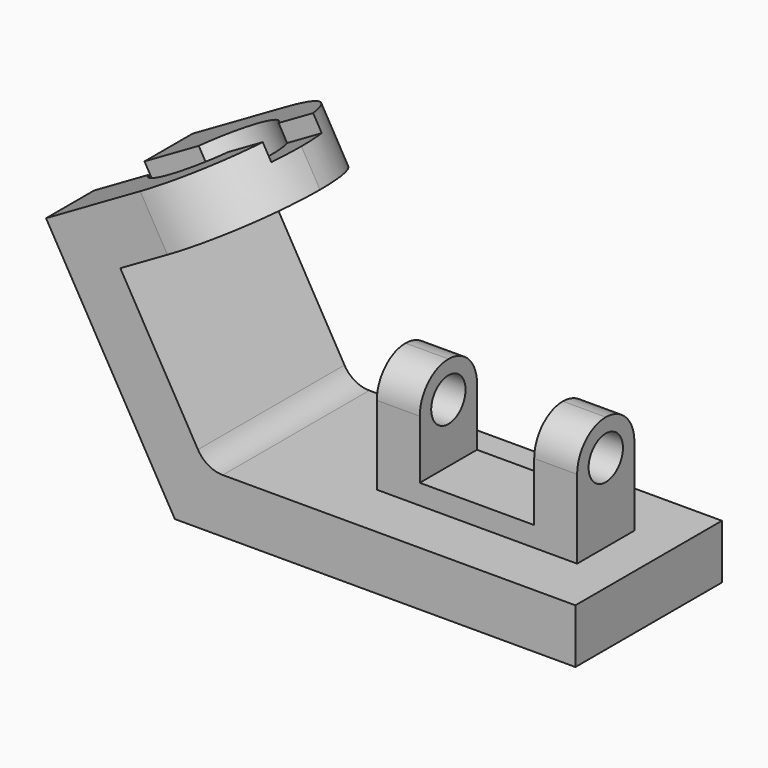
from build123d import *

# Parameters (mm, degrees)
F1_DEPTH  = 32
F2_DEPTH  = 12.5
F4_DEPTH  = 19
F5_R      = 10
F6_R      = 5
F7_DEPTH  = 19
F6_R_2    = 19.5
F8_DEPTH  = 12
F10_DEPTH = 6
F11_W     = 22
F11_H     = 56
F12_DEPTH = 6
F14_DEPTH = 70
F15_R     = 7.5
F16_DEPTH = 70


with BuildPart() as f1:
    # F0 (on Front) → F1 (new body, symmetric)
    with BuildSketch(Plane.XZ):
        Polygon((-45, 77.9422863406), (0, 0), (140, 0), (140, 19), (125, 19), (55, 19), (10.9696551146, 19), (-19.0455173281, 70.9878036687), (25.1217782649, 96.4878036687), (15.6217782649, 112.9422863406), align=None)
    extrude(amount=F1_DEPTH, both=True)

    # F0 (on Front) → F2 (join, symmetric)
    with BuildSketch(Plane.XZ):
        Polygon((55, 19), (125, 19), (125, 59), (110, 59), (110, 26), (70, 26), (70, 59), (55, 59), align=None)
    extrude(amount=F2_DEPTH, both=True)

    # F3 (on face) → F4 (cut, through all)
    with BuildSketch(Plane(origin=(-45, 0, 77.9422863406), x_dir=(0.8660254038, 0, 0.5), z_dir=(-0.5, 0, 0.8660254038))):
        with BuildLine():
            ThreePointArc((38, 32), (60.627416998, 22.627416998), (70, 0))
            Line((70, 0), (70, 32))
            Line((70, 32), (38, 32))
        make_face()
        with BuildLine():
            Line((70, -32), (70, 0))
            ThreePointArc((70, 0), (60.627416998, -22.627416998), (38, -32))
            Line((38, -32), (70, -32))
        make_face()
    extrude(amount=-F4_DEPTH, mode=Mode.SUBTRACT)

    # F5
    f5_edges = [f1.edges().sort_by_distance(p)[0] for p in [
        (10.969655, 0, 19),
    ]]
    fillet(f5_edges, radius=F5_R)

    # F6 (on face) → F7 (cut, through all)
    with BuildSketch(Plane(origin=(-45, 0, 77.9422863406), x_dir=(0.8660254038, 0, 0.5), z_dir=(-0.5, 0, 0.8660254038))):
        with Locations((38, 0)):
            Circle(F6_R)
    extrude(amount=-F7_DEPTH, mode=Mode.SUBTRACT)

    # F6 (on face) → F8 (cut)
    with BuildSketch(Plane(origin=(-45, 0, 77.9422863406), x_dir=(0.8660254038, 0, 0.5), z_dir=(-0.5, 0, 0.8660254038))):
        with Locations((38, 0)):
            Circle(F6_R_2)
        with Locations((38, 0)):
            Circle(F6_R, mode=Mode.SUBTRACT)
    extrude(amount=-F8_DEPTH, mode=Mode.SUBTRACT)

    # F9 (on face) → F10 (cut)
    with BuildSketch(Plane(origin=(-45, 0, 77.9422863406), x_dir=(0.8660254038, 0, 0.5), z_dir=(-0.5, 0, 0.8660254038))):
        with BuildLine():
            Line((21.8987578119, 11), (0, 11))
            Line((0, 11), (0, -11))
            Line((0, -11), (21.8987578119, -11))
            ThreePointArc((21.8987578119, -11), (18.5, 0), (21.8987578119, 11))
        make_face()
        with BuildLine():
            Line((68.0499584026, 11), (54.1012421881, 11))
            ThreePointArc((54.1012421881, 11), (56.630944993, 5.7565518035), (57.5, 0))
            ThreePointArc((57.5, 0), (56.630944993, -5.7565518035), (54.1012421881, -11))
            Line((54.1012421881, -11), (68.0499584026, -11))
            ThreePointArc((68.0499584026, -11), (70, 0), (68.0499584026, 11))
        make_face()
    extrude(amount=-F10_DEPTH, mode=Mode.SUBTRACT)

    # F11 (on face) → F12 (cut)
    with BuildSketch(Plane(origin=(0, 0, 0), x_dir=(0, -1, 0), z_dir=(-0.8660254038, 0, -0.5))):
        with Locations((0, 56)):
            Rectangle(F11_W, F11_H)
    extrude(amount=-F12_DEPTH, mode=Mode.SUBTRACT)

    # F13 (on face) → F14 (cut, through all)
    with BuildSketch(Plane.YZ.offset(125)):
        with BuildLine():
            ThreePointArc((-12.5, 46.5), (-8.8388347372, 55.3388347924), (7.81e-08, 59))
            Line((7.81e-08, 59), (-12.5, 59))
            Line((-12.5, 59), (-12.5, 46.5))
        make_face()
        with BuildLine():
            ThreePointArc((7.81e-08, 59), (8.8388347924, 55.3388347372), (12.5, 46.5))
            Line((12.5, 46.5), (12.5, 59))
            Line((12.5, 59), (7.81e-08, 59))
        make_face()
    extrude(amount=-F14_DEPTH, mode=Mode.SUBTRACT)

    # F15 (on face) → F16 (cut, through all)
    with BuildSketch(Plane.YZ.offset(125)):
        with Locations((0, 46.5)):
            Circle(F15_R)
    extrude(amount=-F16_DEPTH, mode=Mode.SUBTRACT)


solid = f1.part
